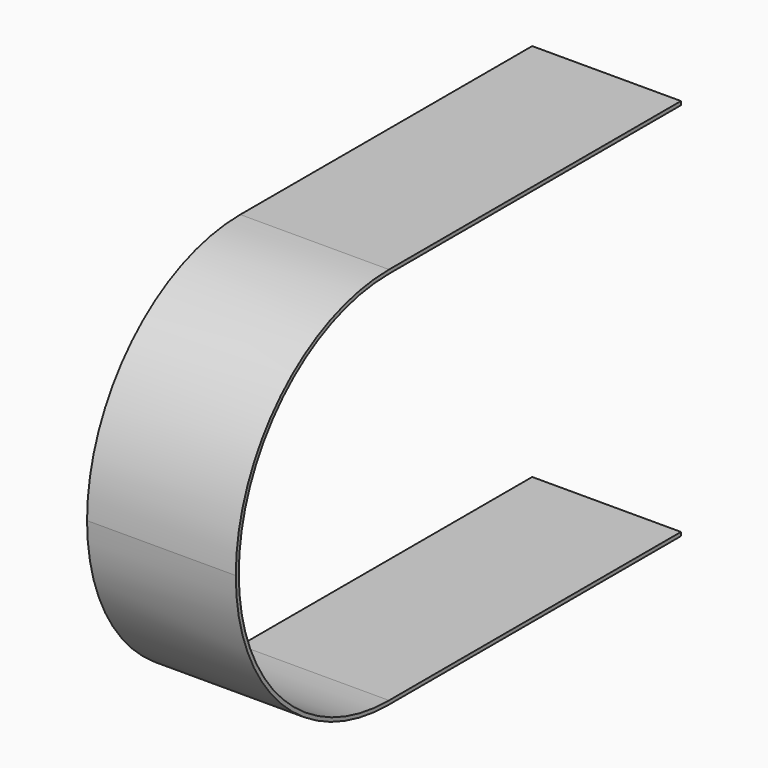
from build123d import *

# Parameters (mm, degrees)
F4_DEPTH = 20


# Not quite as in the source:
# - a feature of the source that left no trace in its solid (it failed there, or was rolled back) is left out


with BuildPart() as f4:
    # F2 (on Right) → F4 (new body)
    with BuildSketch(Plane.YZ):
        with BuildLine():
            ThreePointArc((-25.25, 0), (-17.854446225, 17.854446225), (0, 25.25))
            Line((0, 25.25), (49.0651577711, 25.25))
            Line((49.0651577711, 25.25), (49.0651577711, 25.75))
            Line((49.0651577711, 25.75), (0, 25.75))
            ThreePointArc((0, 25.75), (-18.2079996156, 18.2079996156), (-25.75, 0))
            Line((-25.75, 0), (-25.25, 0))
        make_face()
        with BuildLine():
            ThreePointArc((0, -25.25), (-17.854446225, -17.854446225), (-25.25, 0))
            Line((-25.25, 0), (-25.75, 0))
            ThreePointArc((-25.75, 0), (-18.2079996156, -18.2079996156), (0, -25.75))
            Line((0, -25.75), (49.0651577711, -25.75))
            Line((49.0651577711, -25.75), (49.0651577711, -25.25))
            Line((49.0651577711, -25.25), (0, -25.25))
        make_face()
    extrude(amount=F4_DEPTH)


solid = f4.part
